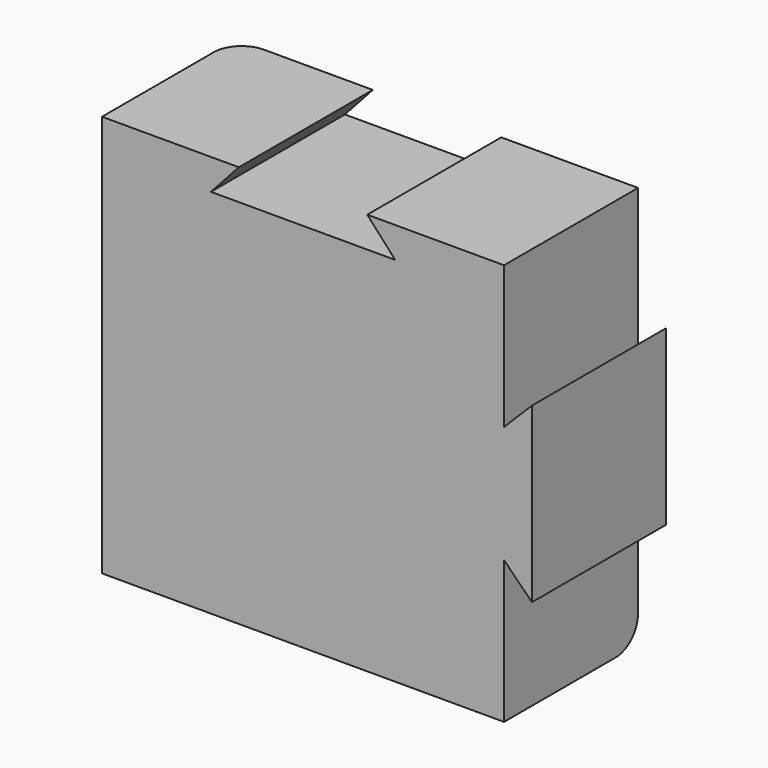
from build123d import *

# Parameters (mm, degrees)
F0_W     = 2
F0_H     = 10
F1_DEPTH = 40
F2_W     = 50
F2_H     = 30
F3_DEPTH = 5
F4_W     = 50
F4_H     = 30
F5_DEPTH = 5
F6_W     = 50
F6_H     = 50
F7_DEPTH = 30
F8_R     = 5
F9_R     = 5


# Not quite as in the source:
# - a feature names something its author has since deleted; it is built from what else it names


with BuildPart() as f1:
    # F0 (on Top) → F1 (new body)
    with BuildSketch(Plane.XY):
        with Locations((-24, 5)):
            Rectangle(F0_W, F0_H)
        with Locations((24, 5)):
            Rectangle(F0_W, F0_H)
        Polygon((-25, 0), (-25, -20), (25, -20), (25, 0), (23, 0), (20, 0), (20, -15), (-20, -15), (-20, 0), (-23, 0), align=None)
    extrude(amount=F1_DEPTH)

    # F2 (on face) → F3 (join)
    with BuildSketch(Plane.XY.offset(40)):
        with Locations((0, -5)):
            Rectangle(F2_W, F2_H)
    extrude(amount=F3_DEPTH)

    # F4 (on face) → F5 (join)
    with BuildSketch(Plane(origin=(0, 0, 0), x_dir=(1, 0, 0), z_dir=(0, 0, -1))):
        with Locations((0, 5)):
            Rectangle(F4_W, F4_H)
    extrude(amount=F5_DEPTH)

    # F6 (on face) → F7 (join)
    with BuildSketch(Plane(origin=(0, 10, 0), x_dir=(-1, 0, 0), z_dir=(0, 1, 0))):
        Polygon((-36, 9.5), (-36, -16), (36, -16), (36, 56), (11.5, 56), (16.5, 50.5), (-16.5, 50.5), (-11.5, 56), (-36, 56), (-36, 30.5), align=None)
        with Locations((0, 20)):
            Rectangle(F6_W, F6_H, mode=Mode.SUBTRACT)
        Polygon((-41, 4.5), (-36, 9.5), (-36, 30.5), (-41, 35.5), align=None)
    extrude(amount=-F7_DEPTH)

    # F8
    f8_edges = [f1.edges().sort_by_distance(p)[0] for p in [
        (0, 10, 0),
        (23, 10, 20),
        (0, 10, 40),
        (-23, 10, 20),
        (-36, 10, 20),
        (0, 10, -16),
    ]]
    fillet(f8_edges, radius=F8_R)

    # F9
    f9_edges = [f1.edges().sort_by_distance(p)[0] for p in [
        (20, -15, 20),
        (0, -15, 0),
        (0, -15, 40),
        (-20, -15, 20),
    ]]
    fillet(f9_edges, radius=F9_R)


solid = f1.part
